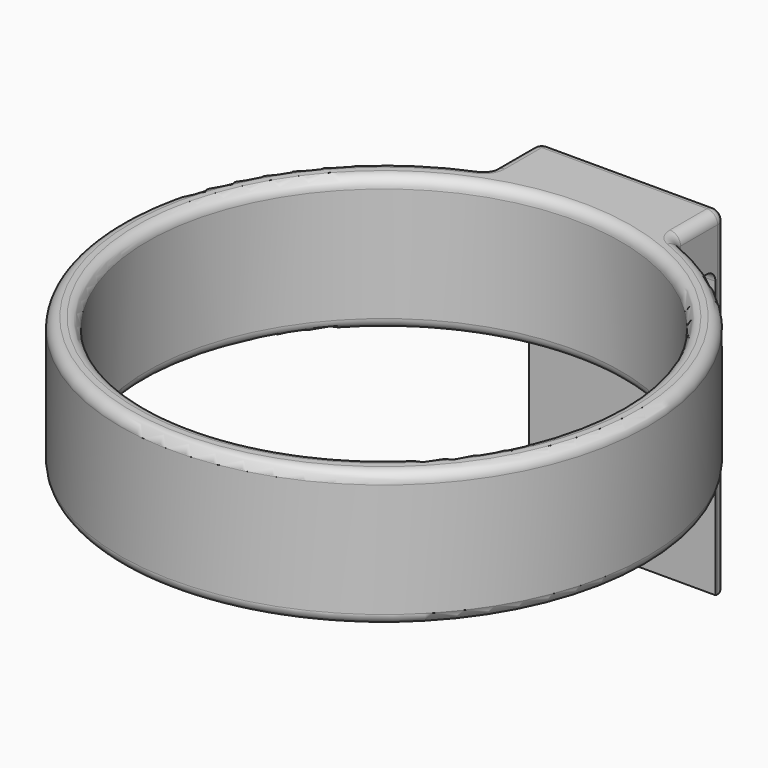
from build123d import *

# Parameters (mm, degrees)
F0_R     = 49.53
F0_R_2   = 44.45
F1_DEPTH = 25.4
F3_DEPTH = 17.5
F4_R     = 2


with BuildPart() as f1:
    # F0 (on Top) → F1 (new body)
    with BuildSketch(Plane.XY):
        Circle(F0_R)
        Circle(F0_R_2, mode=Mode.SUBTRACT)
    extrude(amount=F1_DEPTH)

    # F2 (on Right) → F3 (join, symmetric)
    with BuildSketch(Plane.YZ):
        Polygon((58.382712847, 25.4), (45.682712847, 25.4), (45.682712847, 16.2404105067), (55.88, 16.2404105067), (55.88, -37.6108922064), (58.382712847, -38.1), align=None)
    extrude(amount=F3_DEPTH, both=True)

    # F4
    f4_edges = [f1.edges().sort_by_distance(p)[0] for p in [
        (0, 55.88, 16.240411),
        (0, 49.53, 16.240411),
        (17.5, 46.335417, 20.820205),
        (-17.5, 46.335417, 20.820205),
        (0, 58.382713, 25.4),
        (-44.45, 0, 25.4),
        (-49.53, 0, 0),
        (49.53, 0, 12.7),
        (-28.164214, -40.743072, 25.4),
        (40.743072, 28.164214, 25.4),
        (44.45, 0, 12.7),
        (-44.45, 0, 0),
        (-17.5, 58.382713, -6.35),
        (17.5, 58.382713, -6.35),
        (0, 58.382713, -38.1),
        (17.5, 52.359065, 25.4),
        (-17.5, 52.359065, 25.4),
    ]]
    fillet(f4_edges, radius=F4_R)


solid = f1.part
